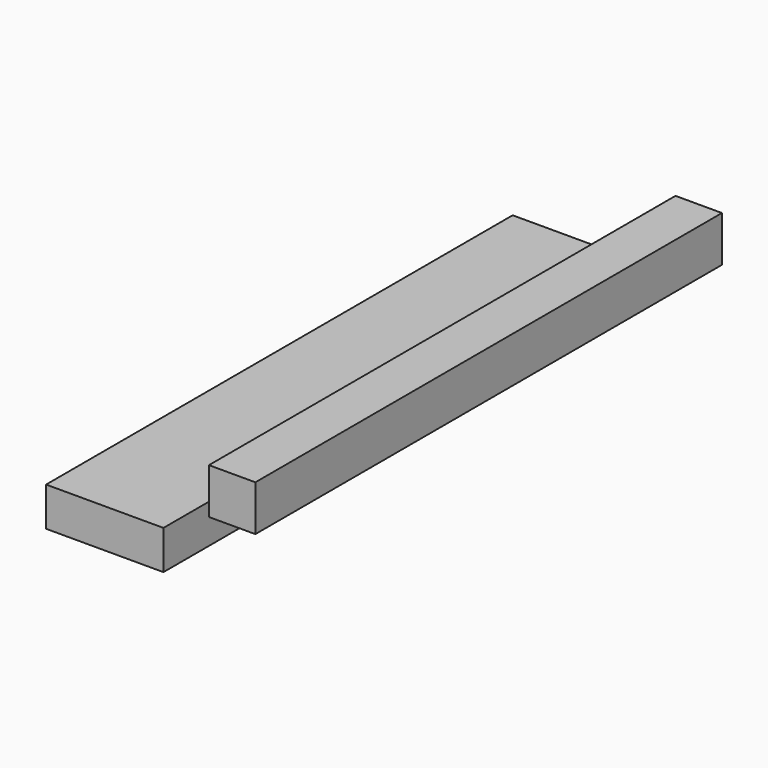
from build123d import *

# Parameters (mm, degrees)
F0_W     = 97.1144884825
F0_H     = 32.2388261557
F1_DEPTH = 241.3


# Not quite as in the source:
# - the program builds the solid bodies; features that only make, move or delete a surface that nothing else refers to are left out


with BuildPart() as f1:
    # F0 (on Front) → F1 (new body, symmetric)
    with BuildSketch(Plane.XZ):
        Rectangle(F0_W, F0_H)
    extrude(amount=F1_DEPTH, both=True)


with BuildPart() as f1b:
    # F0 (on Front) → F1, piece 2 (new body, symmetric)
    with BuildSketch(Plane.XZ):
        Polygon((86.1985152434, 74.0841701627), (86.1985152434, 55.1967807114), (86.1985152434, 36.3093912601), (124.6246164511, 36.3093912601), (124.6246164511, 74.0841701627), align=None)
    extrude(amount=F1_DEPTH, both=True)


solid = Compound([f1.part, f1b.part])
